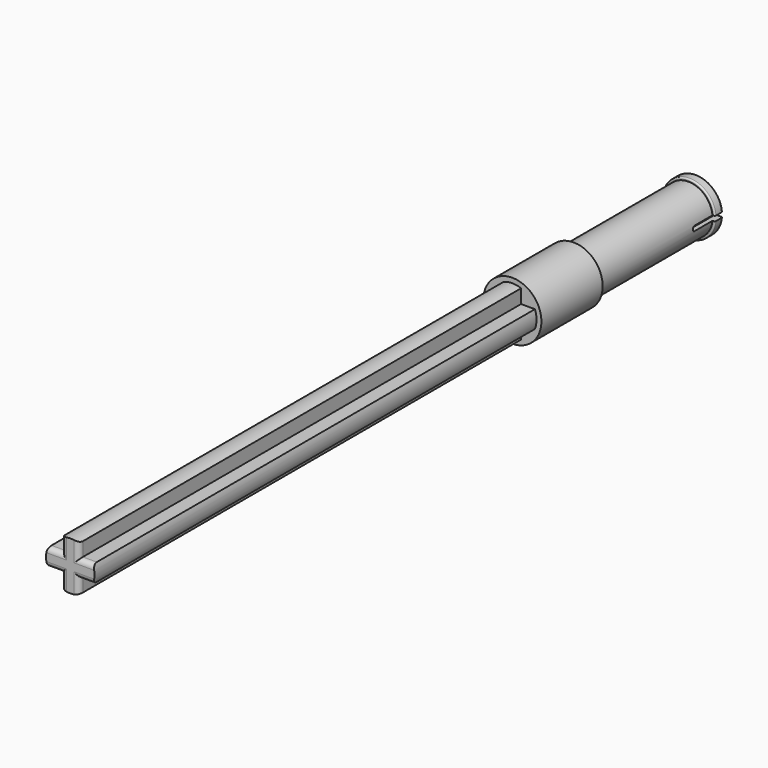
from build123d import *

# Parameters (mm, degrees)
F1_DEPTH  = 28.5
F2_R      = 0.5
F3_R      = 3
F4_DEPTH  = 7.9
F5_R      = 2.499
F5_R_2    = 1.999
F6_DEPTH  = 14.8
F7_R      = 2.75
F7_R_2    = 2.499
F7_R_3    = 1.999
F8_DEPTH  = 1
F10_DEPTH = 3.5
F11_R     = 0.15
F12_R     = 0.15


# Not quite as in the source:
# - a feature names something its author has since deleted; it is built from what else it names


with BuildPart() as f1:
    # F0 (on Front) → F1 (new body, symmetric)
    with BuildSketch(Plane.XZ):
        with BuildLine():
            Line((-0.9, 0.9), (-2.3313088598, 0.9))
            ThreePointArc((-2.3313088598, 0.9), (-2.499, 0), (-2.3313088598, -0.9))
            Line((-2.3313088598, -0.9), (-0.9, -0.9))
            Line((-0.9, -0.9), (-0.9, -2.3313088598))
            ThreePointArc((-0.9, -2.3313088598), (0, -2.499), (0.9, -2.3313088598))
            Line((0.9, -2.3313088598), (0.9, -0.9))
            Line((0.9, -0.9), (2.3313088598, -0.9))
            ThreePointArc((2.3313088598, -0.9), (2.499, 0), (2.3313088598, 0.9))
            Line((2.3313088598, 0.9), (0.9, 0.9))
            Line((0.9, 0.9), (0.9, 2.3313088598))
            ThreePointArc((0.9, 2.3313088598), (0, 2.499), (-0.9, 2.3313088598))
            Line((-0.9, 2.3313088598), (-0.9, 0.9))
        make_face()
    extrude(amount=F1_DEPTH, both=True)

    # F2
    f2_edges = [f1.edges().sort_by_distance(p)[0] for p in [
        (0.9, -28.5, 1.615654),
        (-0.9, -28.5, 1.615654),
        (1.615654, -28.5, 0.9),
        (1.615654, -28.5, -0.9),
        (0.9, -28.5, -1.615654),
        (-0.9, -28.5, -1.615654),
        (-1.615654, -28.5, -0.9),
        (-1.615654, -28.5, 0.9),
    ]]
    fillet(f2_edges, radius=F2_R)

    # F3 (on face) → F4 (join)
    with BuildSketch(Plane(origin=(0, 28.5, 0), x_dir=(-1, 0, 0), z_dir=(0, 1, 0))):
        Circle(F3_R)
        with BuildLine():
            Line((-2.3313088598, 0.9), (-0.9, 0.9))
            Line((-0.9, 0.9), (-0.9, 2.3313088598))
            ThreePointArc((-0.9, 2.3313088598), (0, 2.499), (0.9, 2.3313088598))
            Line((0.9, 2.3313088598), (0.9, 0.9))
            Line((0.9, 0.9), (2.3313088598, 0.9))
            ThreePointArc((2.3313088598, 0.9), (2.499, 0), (2.3313088598, -0.9))
            Line((2.3313088598, -0.9), (0.9, -0.9))
            Line((0.9, -0.9), (0.9, -2.3313088598))
            ThreePointArc((0.9, -2.3313088598), (0, -2.499), (-0.9, -2.3313088598))
            Line((-0.9, -2.3313088598), (-0.9, -0.9))
            Line((-0.9, -0.9), (-2.3313088598, -0.9))
            ThreePointArc((-2.3313088598, -0.9), (-2.499, 0), (-2.3313088598, 0.9))
        make_face(mode=Mode.SUBTRACT)
        with BuildLine():
            Line((-0.9, 2.3313088598), (-0.9, 0.9))
            Line((-0.9, 0.9), (-2.3313088598, 0.9))
            ThreePointArc((-2.3313088598, 0.9), (-2.499, 0), (-2.3313088598, -0.9))
            Line((-2.3313088598, -0.9), (-0.9, -0.9))
            Line((-0.9, -0.9), (-0.9, -2.3313088598))
            ThreePointArc((-0.9, -2.3313088598), (0, -2.499), (0.9, -2.3313088598))
            Line((0.9, -2.3313088598), (0.9, -0.9))
            Line((0.9, -0.9), (2.3313088598, -0.9))
            ThreePointArc((2.3313088598, -0.9), (2.499, 0), (2.3313088598, 0.9))
            Line((2.3313088598, 0.9), (0.9, 0.9))
            Line((0.9, 0.9), (0.9, 2.3313088598))
            ThreePointArc((0.9, 2.3313088598), (0, 2.499), (-0.9, 2.3313088598))
        make_face()
    extrude(amount=F4_DEPTH)

    # F5 (on face) → F6 (join)
    with BuildSketch(Plane(origin=(0, 36.4, 0), x_dir=(-1, 0, 0), z_dir=(0, 1, 0))):
        Circle(F5_R)
        Circle(F5_R_2, mode=Mode.SUBTRACT)
    extrude(amount=F6_DEPTH)

    # F7 (on face) → F8 (join)
    with BuildSketch(Plane(origin=(0, 51.2, 0), x_dir=(-1, 0, 0), z_dir=(0, 1, 0))):
        Circle(F7_R)
        Circle(F7_R_2, mode=Mode.SUBTRACT)
        Circle(F7_R_2)
        Circle(F7_R_3, mode=Mode.SUBTRACT)
    extrude(amount=F8_DEPTH)

    # F9 (on face) → F10 (cut)
    with BuildSketch(Plane(origin=(0, 52.2, 0), x_dir=(-1, 0, 0), z_dir=(0, 1, 0))):
        with BuildLine():
            ThreePointArc((-1.983305574, -0.25), (-1.999, 0), (-1.983305574, 0.25))
            Line((-1.983305574, 0.25), (-2.7386127875, 0.25))
            ThreePointArc((-2.7386127875, 0.25), (-2.75, 0), (-2.7386127875, -0.25))
            Line((-2.7386127875, -0.25), (-1.983305574, -0.25))
        make_face()
        with BuildLine():
            ThreePointArc((2.7386127875, -0.25), (2.75, 0), (2.7386127875, 0.25))
            Line((2.7386127875, 0.25), (1.983305574, 0.25))
            ThreePointArc((1.983305574, 0.25), (1.999, 0), (1.983305574, -0.25))
            Line((1.983305574, -0.25), (2.7386127875, -0.25))
        make_face()
    extrude(amount=-F10_DEPTH, mode=Mode.SUBTRACT)

    # F11
    f11_edges = [f1.edges().sort_by_distance(p)[0] for p in [
        (2.234885, 48.7, -0.25),
        (2.234885, 48.7, 0.25),
        (-2.234885, 48.7, -0.25),
        (-2.234885, 48.7, 0.25),
    ]]
    fillet(f11_edges, radius=F11_R)

    # F12
    f12_edges = [f1.edges().sort_by_distance(p)[0] for p in [
        (0, 52.2, 2.75),
        (0, 52.2, -2.75),
        (0, 51.2, -2.75),
        (0, 51.2, 2.75),
    ]]
    fillet(f12_edges, radius=F12_R)


solid = f1.part
